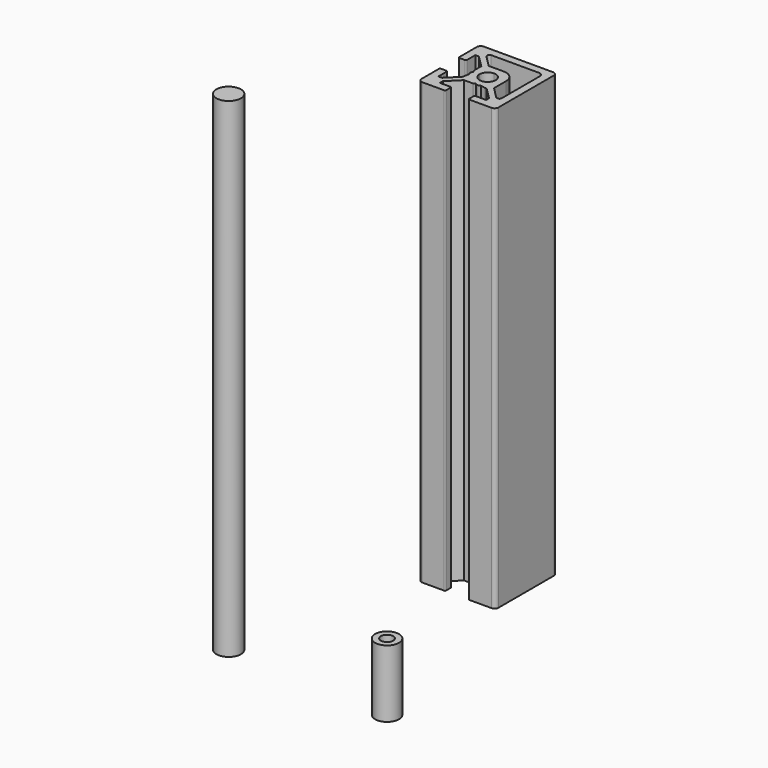
from build123d import *

# Parameters (mm, degrees)
F0_R     = 3.175
F1_DEPTH = 127
F3_DEPTH = 114.3
F0_R_2   = 3.1
F0_R_3   = 1.6
F4_DEPTH = 17.4625


# Not quite as in the source:
# - ends of sketch curves that miss each other by under 0.0002 mm in the source are joined
# - a length typed as a fraction of an inch, garbled in the dataset ("3 / 203.2 mm" for 3/8 in), is restored


with BuildPart() as f1:
    # F0 (on Top) → F1 (new body)
    with BuildSketch(Plane.XY):
        with Locations((-56.0373365879, -48.2565127313)):
            Circle(F0_R)
    extrude(amount=F1_DEPTH)


with BuildPart() as f3:
    # F2 (on Top) → F3 (new body)
    with BuildSketch(Plane.XY):
        with BuildLine():
            Line((-34.856435, 17.273321), (-34.856435, 19.273321))
            Line((-34.856435, 19.273321), (-43.856435, 19.273321))
            ThreePointArc((-43.856435, 19.273321), (-44.5635417812, 18.9804277812), (-44.856435, 18.273321))
            Line((-44.856435, 18.273321), (-44.856435, 12.573321))
            ThreePointArc((-44.856435, 12.573321), (-44.7685670344, 12.3611889656), (-44.556435, 12.273321))
            Line((-44.556435, 12.273321), (-43.156435, 12.273321))
            ThreePointArc((-43.156435, 12.273321), (-42.9443029656, 12.3611889656), (-42.856435, 12.573321))
            Line((-42.856435, 12.573321), (-42.856435, 15.273321))
            Line((-42.856435, 15.273321), (-41.917095, 15.273321))
            Line((-41.917095, 15.273321), (-38.856435, 12.212661))
            Line((-38.856435, 12.212661), (-38.856435, 9.926911))
            ThreePointArc((-38.856435, 9.926911), (-38.8393979324, 9.7975015494), (-38.7894477764, 9.6769111291))
            Line((-38.7894477764, 9.6769111291), (-38.556435, 9.273321))
            Line((-38.556435, 9.273321), (-36.956435, 9.273321))
            ThreePointArc((-36.956435, 9.273321), (-36.3413592405, 10.7582452405), (-34.856435, 11.373321))
            Line((-34.856435, 11.373321), (-34.856435, 13.273321))
            Line((-34.856435, 13.273321), (-37.588668, 13.273321))
            ThreePointArc((-37.588668, 13.273321), (-37.7800097162, 13.3113812337), (-37.9422213906, 13.4197676094))
            Line((-37.9422213906, 13.4197676094), (-40.709988, 16.187535))
            ThreePointArc((-40.709988, 16.187535), (-40.8183747663, 16.3497462838), (-40.856435, 16.541088))
            Line((-40.856435, 16.541088), (-40.856435, 16.773321))
            ThreePointArc((-40.856435, 16.773321), (-40.7099883906, 17.1268743906), (-40.356435, 17.273321))
            Line((-40.356435, 17.273321), (-34.856435, 17.273321))
        make_face()
        with BuildLine():
            Line((-25.856435, 19.273321), (-34.856435, 19.273321))
            Line((-34.856435, 19.273321), (-34.856435, 17.273321))
            Line((-34.856435, 17.273321), (-27.856435, 17.273321))
            ThreePointArc((-27.856435, 17.273321), (-27.1493282188, 16.9804277812), (-26.856435, 16.273321))
            Line((-26.856435, 16.273321), (-26.856435, 9.273321))
            Line((-26.856435, 9.273321), (-24.856435, 9.273321))
            Line((-24.856435, 9.273321), (-24.856435, 18.273321))
            ThreePointArc((-24.856435, 18.273321), (-25.1493282188, 18.9804277812), (-25.856435, 19.273321))
        make_face()
        with BuildLine():
            Line((-24.856435, 0.273321), (-24.856435, 9.273321))
            Line((-24.856435, 9.273321), (-26.856435, 9.273321))
            Line((-26.856435, 9.273321), (-26.856435, 3.773321))
            ThreePointArc((-26.856435, 3.773321), (-27.0028816094, 3.4197676094), (-27.356435, 3.273321))
            Line((-27.356435, 3.273321), (-27.588668, 3.273321))
            ThreePointArc((-27.588668, 3.273321), (-27.7800097162, 3.3113812337), (-27.9422213906, 3.4197676094))
            Line((-27.9422213906, 3.4197676094), (-30.709988, 6.187535))
            ThreePointArc((-30.709988, 6.187535), (-30.8183747663, 6.3497462838), (-30.856435, 6.541088))
            Line((-30.856435, 6.541088), (-30.856435, 9.273321))
            Line((-30.856435, 9.273321), (-32.756435, 9.273321))
            ThreePointArc((-32.756435, 9.273321), (-33.3715107595, 7.7883967595), (-34.856435, 7.173321))
            Line((-34.856435, 7.173321), (-34.856435, 5.573321))
            Line((-34.856435, 5.573321), (-34.452845, 5.340308))
            ThreePointArc((-34.452845, 5.340308), (-34.202845, 5.273321), (-33.9528451291, 5.3403082236))
            Line((-33.9528451291, 5.3403082236), (-33.637549, 5.522344))
            Line((-33.637549, 5.522344), (-32.356435, 5.273321))
            Line((-32.356435, 5.273321), (-31.917095, 5.273321))
            Line((-31.917095, 5.273321), (-28.856435, 2.212661))
            Line((-28.856435, 2.212661), (-28.856435, 1.273321))
            Line((-28.856435, 1.273321), (-31.556435, 1.273321))
            ThreePointArc((-31.556435, 1.273321), (-31.7685670344, 1.1854530344), (-31.856435, 0.973321))
            Line((-31.856435, 0.973321), (-31.856435, -0.426679))
            ThreePointArc((-31.856435, -0.426679), (-31.7685670344, -0.6388110344), (-31.556435, -0.726679))
            Line((-31.556435, -0.726679), (-25.856435, -0.726679))
            ThreePointArc((-25.856435, -0.726679), (-25.1493282188, -0.4337857812), (-24.856435, 0.273321))
        make_face()
        with BuildLine():
            Line((-33.856435, 13.273321), (-34.856435, 13.273321))
            Line((-34.856435, 13.273321), (-34.856435, 11.373321))
            ThreePointArc((-34.856435, 11.373321), (-33.3715107595, 10.7582452405), (-32.756435, 9.273321))
            Line((-32.756435, 9.273321), (-30.856435, 9.273321))
            Line((-30.856435, 9.273321), (-30.856435, 10.273321))
            ThreePointArc((-30.856435, 10.273321), (-31.7351146564, 12.3946413436), (-33.856435, 13.273321))
        make_face()
        with BuildLine():
            ThreePointArc((-34.856435, 7.173321), (-36.3413592405, 7.7883967595), (-36.956435, 9.273321))
            Line((-36.956435, 9.273321), (-38.556435, 9.273321))
            Line((-38.556435, 9.273321), (-38.789448, 8.869731))
            ThreePointArc((-38.789448, 8.869731), (-38.856435, 8.619731), (-38.7894477764, 8.3697311291))
            Line((-38.7894477764, 8.3697311291), (-38.607412, 8.054435))
            Line((-38.607412, 8.054435), (-38.856435, 6.773321))
            Line((-38.856435, 6.773321), (-38.856435, 6.333981))
            Line((-38.856435, 6.333981), (-41.917095, 3.273321))
            Line((-41.917095, 3.273321), (-42.856435, 3.273321))
            Line((-42.856435, 3.273321), (-42.856435, 5.973321))
            ThreePointArc((-42.856435, 5.973321), (-42.9443029656, 6.1854530344), (-43.156435, 6.273321))
            Line((-43.156435, 6.273321), (-44.556435, 6.273321))
            ThreePointArc((-44.556435, 6.273321), (-44.7685670344, 6.1854530344), (-44.856435, 5.973321))
            Line((-44.856435, 5.973321), (-44.856435, 0.273321))
            ThreePointArc((-44.856435, 0.273321), (-44.5635417812, -0.4337857812), (-43.856435, -0.726679))
            Line((-43.856435, -0.726679), (-38.156435, -0.726679))
            ThreePointArc((-38.156435, -0.726679), (-37.9443029656, -0.6388110344), (-37.856435, -0.426679))
            Line((-37.856435, -0.426679), (-37.856435, 0.973321))
            ThreePointArc((-37.856435, 0.973321), (-37.9443029656, 1.1854530344), (-38.156435, 1.273321))
            Line((-38.156435, 1.273321), (-40.856435, 1.273321))
            Line((-40.856435, 1.273321), (-40.856435, 2.212661))
            Line((-40.856435, 2.212661), (-37.795775, 5.273321))
            Line((-37.795775, 5.273321), (-35.510025, 5.273321))
            ThreePointArc((-35.510025, 5.273321), (-35.3806155494, 5.2903580676), (-35.2600251291, 5.3403082236))
            Line((-35.2600251291, 5.3403082236), (-34.856435, 5.573321))
            Line((-34.856435, 5.573321), (-34.856435, 7.173321))
        make_face()
    extrude(amount=F3_DEPTH)


with BuildPart() as f4:
    # F0 (on Top) → F4 (new body)
    with BuildSketch(Plane.XY):
        with Locations((-13.1225734949, -50.5226738751)):
            Circle(F0_R_2)
        with Locations((-13.1225734949, -50.5226738751)):
            Circle(F0_R_3, mode=Mode.SUBTRACT)
    extrude(amount=F4_DEPTH)


solid = Compound([f1.part, f3.part, f4.part])
